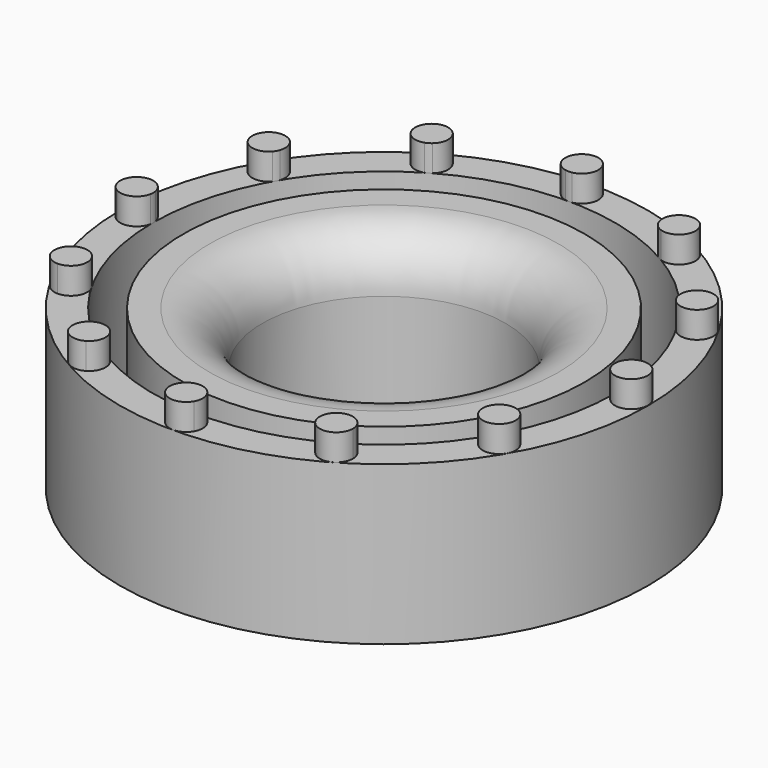
from build123d import *

# Parameters (mm, degrees)
F0_R     = 10
F0_R_2   = 8.75
F1_DEPTH = 6
F0_R_3   = 7.6
F0_R_4   = 4.6
F2_DEPTH = 1
F4_DEPTH = 1
F5_COUNT = 12
F6_R     = 2


with BuildPart() as f1:
    # F0 (on Top) → F1 (new body)
    with BuildSketch(Plane.XY):
        Circle(F0_R)
        Circle(F0_R_2, mode=Mode.SUBTRACT)
    extrude(amount=F1_DEPTH)


with BuildPart() as f1b:
    # F0 (on Top) → F1, piece 2 (new body)
    with BuildSketch(Plane.XY):
        Circle(F0_R_3)
        Circle(F0_R_4, mode=Mode.SUBTRACT)
    extrude(amount=F1_DEPTH)

    # F6
    f6_edges = [f1b.edges().sort_by_distance(p)[0] for p in [
        (-4.6, 0, 6),
    ]]
    fillet(f6_edges, radius=F6_R)


with BuildPart() as f2:
    # F0 (on Top) → F2 (new body)
    with BuildSketch(Plane.XY):
        Circle(F0_R_2)
        Circle(F0_R_3, mode=Mode.SUBTRACT)
    extrude(amount=F2_DEPTH)


with BuildPart() as f4:
    # F3 (on face) → F4 (new body)
    with BuildSketch(Plane.XY.offset(6)):
        with BuildLine():
            ThreePointArc((4.2704616884, -7.6371236056), (4.375, -7.5777222831), (4.4787122101, -7.5168901109))
            ThreePointArc((4.4787122101, -7.5168901109), (4.36875, -7.5668969656), (4.2704616884, -7.6371236056))
        make_face()
        with BuildLine():
            ThreePointArc((5.30625, -8.1081628429), (5.0445947958, -7.5996300914), (4.4787122101, -7.5168901109))
            ThreePointArc((4.4787122101, -7.5168901109), (4.375, -7.5777222831), (4.2704616884, -7.6371236056))
            ThreePointArc((4.2704616884, -7.6371236056), (4.4225201165, -8.6770950422), (5.30625, -8.1081628429))
        make_face()
    extrude(amount=F4_DEPTH)


with BuildPart() as f5_1:
    # F5: instance of F4
    add(f4.part.rotate(Axis((0, 0, 6), (0, 0, 1)), 1 * 360 / F5_COUNT))


with BuildPart() as f5_2:
    # F5: instance of F4
    add(f4.part.rotate(Axis((0, 0, 6), (0, 0, 1)), 2 * 360 / F5_COUNT))


with BuildPart() as f5_3:
    # F5: instance of F4
    add(f4.part.rotate(Axis((0, 0, 6), (0, 0, 1)), 3 * 360 / F5_COUNT))


with BuildPart() as f5_4:
    # F5: instance of F4
    add(f4.part.rotate(Axis((0, 0, 6), (0, 0, 1)), 4 * 360 / F5_COUNT))


with BuildPart() as f5_5:
    # F5: instance of F4
    add(f4.part.rotate(Axis((0, 0, 6), (0, 0, 1)), 5 * 360 / F5_COUNT))


with BuildPart() as f5_6:
    # F5: instance of F4
    add(f4.part.rotate(Axis((0, 0, 6), (0, 0, 1)), 6 * 360 / F5_COUNT))


with BuildPart() as f5_7:
    # F5: instance of F4
    add(f4.part.rotate(Axis((0, 0, 6), (0, 0, 1)), 7 * 360 / F5_COUNT))


with BuildPart() as f5_8:
    # F5: instance of F4
    add(f4.part.rotate(Axis((0, 0, 6), (0, 0, 1)), 8 * 360 / F5_COUNT))


with BuildPart() as f5_9:
    # F5: instance of F4
    add(f4.part.rotate(Axis((0, 0, 6), (0, 0, 1)), 9 * 360 / F5_COUNT))


with BuildPart() as f5_10:
    # F5: instance of F4
    add(f4.part.rotate(Axis((0, 0, 6), (0, 0, 1)), 10 * 360 / F5_COUNT))


with BuildPart() as f5_11:
    # F5: instance of F4
    add(f4.part.rotate(Axis((0, 0, 6), (0, 0, 1)), 11 * 360 / F5_COUNT))


solid = Compound([f1.part, f1b.part, f2.part, f4.part, f5_1.part, f5_2.part, f5_3.part, f5_4.part, f5_5.part, f5_6.part, f5_7.part, f5_8.part, f5_9.part, f5_10.part, f5_11.part])
